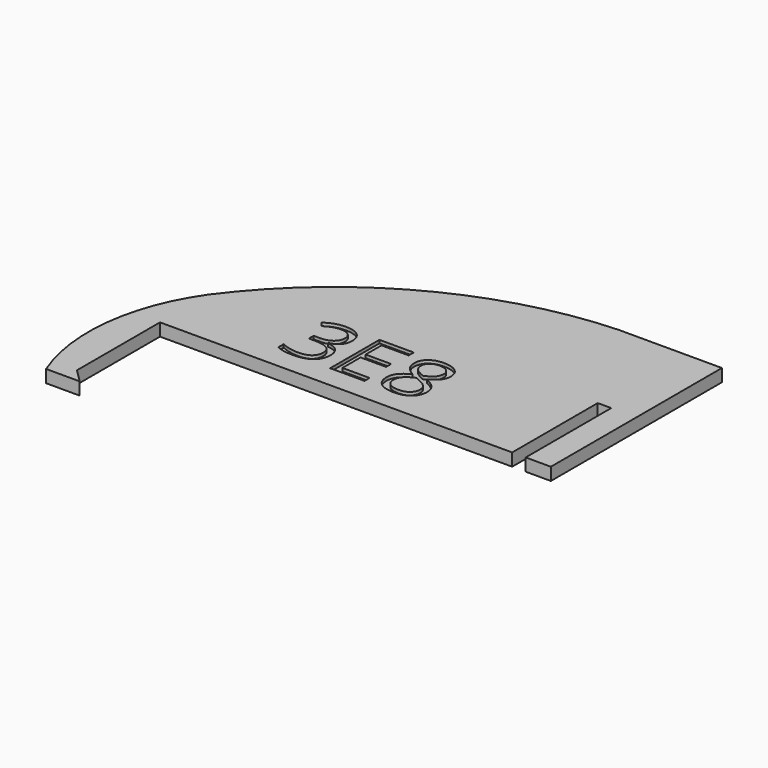
from build123d import *

# Parameters (mm, degrees)
F3_DEPTH     = 2
F4_TEXT_SIZE = 13.7083333333
F5_DEPTH     = 0.5


# Not quite as in the source:
# - Text() gives the source's letters only with a copy of the font that has no kerning and outlines rounded to 1/6400 em; it was checked with that copy


with BuildPart() as f3:
    # F2 (on Top) → F3 (new body)
    with BuildSketch(Plane.XY):
        with BuildLine():
            Line((4.935, -24.13), (4.935, -7.13))
            Line((4.935, -7.13), (7.085, -7.13))
            Line((7.085, -7.13), (7.085, -24.13))
            Line((7.085, -24.13), (11.085, -24.13))
            Line((11.085, -24.13), (11.085, 9.87))
            Line((11.085, 9.87), (0, 9.87))
            Line((0, 9.87), (-5.3746161735, 9.87))
            ThreePointArc((-5.3746161735, 9.87), (-30.9953719156, 2.8325120897), (-51.065, -14.5789608359))
            Line((-51.065, -14.5789608359), (-51.065, -24.13))
            Line((-51.065, -24.13), (4.935, -24.13))
        make_face()
        with BuildLine():
            Line((-51.065, -40.63), (-51.065, -24.13))
            Line((-51.065, -24.13), (-51.065, -14.5789608359))
            ThreePointArc((-51.065, -14.5789608359), (-56.2113850392, -28.2612370174), (-54.2807256494, -42.7513203436))
            Line((-54.2807256494, -42.7513203436), (-48.9436796564, -42.7513203436))
            Line((-48.9436796564, -42.7513203436), (-51.065, -40.63))
        make_face()
    extrude(amount=F3_DEPTH)

    # F4 (on face) → F5 (cut)
    with BuildSketch(Plane.XY.offset(2)):
        with Locations((-36.0380092486, -20.565)):
            Text('3E8', F4_TEXT_SIZE, font='Open Sans', text_align=(TextAlign.LEFT, TextAlign.BOTTOM))
    extrude(amount=-F5_DEPTH, mode=Mode.SUBTRACT)


solid = f3.part
